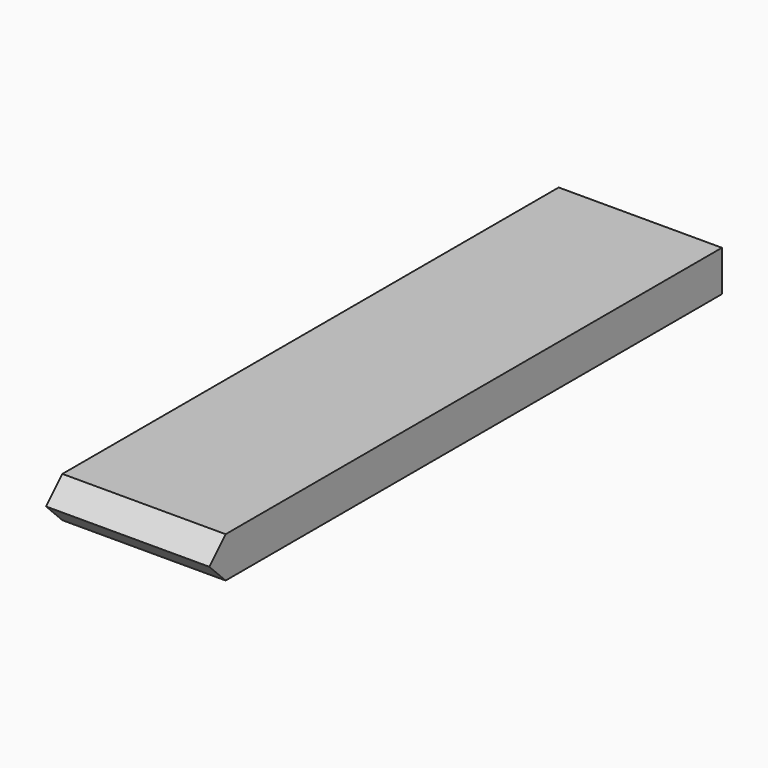
from build123d import *

# Parameters (mm, degrees)
F0_W        = 25.4
F0_H        = 6.35
F1_DEPTH    = 101.6
F2_T1_DEPTH = 51.5282991577


# Not quite as in the source:
# - a fillet or chamfer that OpenCascade refuses, or shapes differently, is made with other operations: its cross-section is extruded or revolved along the edge and cut away or added


with BuildPart() as f1:
    # F0 (on Front) → F1 (new body)
    with BuildSketch(Plane.XZ):
        Rectangle(F0_W, F0_H)
    extrude(amount=F1_DEPTH)

    # F2: chamfer of 5.08 on 2 edges, made by hand

    # F2_s2 → F2_t1 (cut)
    with BuildSketch(Plane.YZ.offset(-25.7641495789)):
        Polygon((-96.52, 3.175), (-101.6, -1.905), (-101.6, 3.175), align=None)
        Polygon((-96.52, -3.175), (-101.6, 1.905), (-101.6, -3.175), align=None)
    extrude(amount=F2_T1_DEPTH, mode=Mode.SUBTRACT)


solid = f1.part
